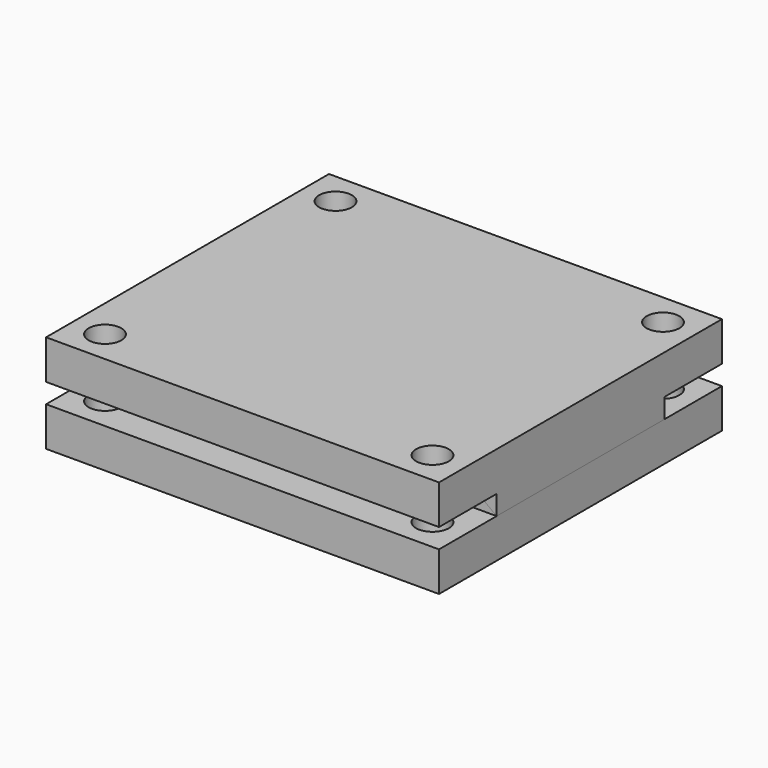
from build123d import *

# Parameters (mm, degrees)
F2_DEPTH = 8
F0_W     = 30
F0_H     = 27
F0_R     = 1.25
F3_DEPTH = 3
F4_DEPTH = 8
F5_START = 1.5
F5_DEPTH = 3


with BuildPart() as f2:
    # F1 (on Front) → F2 (new body, symmetric)
    with BuildSketch(Plane.XZ):
        Polygon((-5, 1.5), (-5, 0), (0, 0), align=None)
        Polygon((-5, 1.5), (-7, 0), (-5, 0), align=None)
    extrude(amount=F2_DEPTH, both=True)



with BuildPart() as f2b:
    # F1 (on Front) → F2, piece 2 (new body, symmetric)
    with BuildSketch(Plane.XZ):
        Polygon((-9, 1.5), (-9, 0), (-7, 0), align=None)
        Polygon((-9, 1.5), (-11, 0), (-9, 0), align=None)
    extrude(amount=F2_DEPTH, both=True)


with BuildPart() as f2c:
    # F1 (on Front) → F2, piece 3 (new body, symmetric)
    with BuildSketch(Plane.XZ):
        Polygon((-13, 1.5), (-13, 0), (-11, 0), align=None)
        Polygon((-13, 1.5), (-15, 0), (-13, 0), align=None)
    extrude(amount=F2_DEPTH, both=True)


with BuildPart() as f2d:
    # F1 (on Front) → F2, piece 4 (new body, symmetric)
    with BuildSketch(Plane.XZ):
        Polygon((5, 1.5), (0, 0), (5, 0), align=None)
        Polygon((7, 0), (5, 1.5), (5, 0), align=None)
    extrude(amount=F2_DEPTH, both=True)


with BuildPart() as f2e:
    # F1 (on Front) → F2, piece 5 (new body, symmetric)
    with BuildSketch(Plane.XZ):
        Polygon((9, 1.5), (7, 0), (9, 0), align=None)
        Polygon((11, 0), (9, 1.5), (9, 0), align=None)
    extrude(amount=F2_DEPTH, both=True)


with BuildPart() as f2f:
    # F1 (on Front) → F2, piece 6 (new body, symmetric)
    with BuildSketch(Plane.XZ):
        Polygon((13, 1.5), (11, 0), (13, 0), align=None)
        Polygon((15, 0), (13, 1.5), (13, 0), align=None)
    extrude(amount=F2_DEPTH, both=True)


with BuildPart() as f2_1:
    add(f2.part)

    add(f2b.part)  # F3 merges F2b

    add(f2c.part)  # F3 merges F2c

    add(f2d.part)  # F3 merges F2d

    add(f2e.part)  # F3 merges F2e

    add(f2f.part)  # F3 merges F2f
    # F0 (on Top) → F3 (join)
    with BuildSketch(Plane.XY):
        Rectangle(F0_W, F0_H)
        with Locations((-12.5, -11)):
            Circle(F0_R, mode=Mode.SUBTRACT)
        with Locations((12.5, -11)):
            Circle(F0_R, mode=Mode.SUBTRACT)
        with Locations((-12.5, 11)):
            Circle(F0_R, mode=Mode.SUBTRACT)
        with Locations((12.5, 11)):
            Circle(F0_R, mode=Mode.SUBTRACT)
    extrude(amount=-F3_DEPTH)


with BuildPart() as f4:
    # F1 (on Front) → F4 (new body, symmetric)
    with BuildSketch(Plane.XZ):
        Polygon((-15, 1.5), (-15, 0), (-13, 1.5), align=None)
    extrude(amount=F4_DEPTH, both=True)

    # F1 (on Front) → F4, piece 2 (join, symmetric)
    with BuildSketch(Plane.XZ):
        Polygon((-11, 1.5), (-13, 1.5), (-11, 0), align=None)
        Polygon((-11, 1.5), (-11, 0), (-9, 1.5), align=None)
    extrude(amount=F4_DEPTH, both=True)

    # F1 (on Front) → F4, piece 3 (join, symmetric)
    with BuildSketch(Plane.XZ):
        Polygon((-7, 1.5), (-9, 1.5), (-7, 0), align=None)
        Polygon((-7, 1.5), (-7, 0), (-5, 1.5), align=None)
    extrude(amount=F4_DEPTH, both=True)

    # F1 (on Front) → F4, piece 4 (join, symmetric)
    with BuildSketch(Plane.XZ):
        Polygon((5, 1.5), (-5, 1.5), (0, 0), align=None)
    extrude(amount=F4_DEPTH, both=True)

    # F1 (on Front) → F4, piece 5 (join, symmetric)
    with BuildSketch(Plane.XZ):
        Polygon((7, 1.5), (5, 1.5), (7, 0), align=None)
        Polygon((9, 1.5), (7, 1.5), (7, 0), align=None)
    extrude(amount=F4_DEPTH, both=True)

    # F1 (on Front) → F4, piece 6 (join, symmetric)
    with BuildSketch(Plane.XZ):
        Polygon((11, 1.5), (9, 1.5), (11, 0), align=None)
        Polygon((13, 1.5), (11, 1.5), (11, 0), align=None)
    extrude(amount=F4_DEPTH, both=True)

    # F1 (on Front) → F4, piece 7 (join, symmetric)
    with BuildSketch(Plane.XZ):
        Polygon((15, 1.5), (13, 1.5), (15, 0), align=None)
    extrude(amount=F4_DEPTH, both=True)

    # F0 (on Top) → F5 (join)
    with BuildSketch(Plane.XY.offset(F5_START)):
        Rectangle(F0_W, F0_H)
        with Locations((-12.5, -11)):
            Circle(F0_R, mode=Mode.SUBTRACT)
        with Locations((12.5, -11)):
            Circle(F0_R, mode=Mode.SUBTRACT)
        with Locations((-12.5, 11)):
            Circle(F0_R, mode=Mode.SUBTRACT)
        with Locations((12.5, 11)):
            Circle(F0_R, mode=Mode.SUBTRACT)
    extrude(amount=F5_DEPTH)


solid = Compound([f2_1.part, f4.part])
